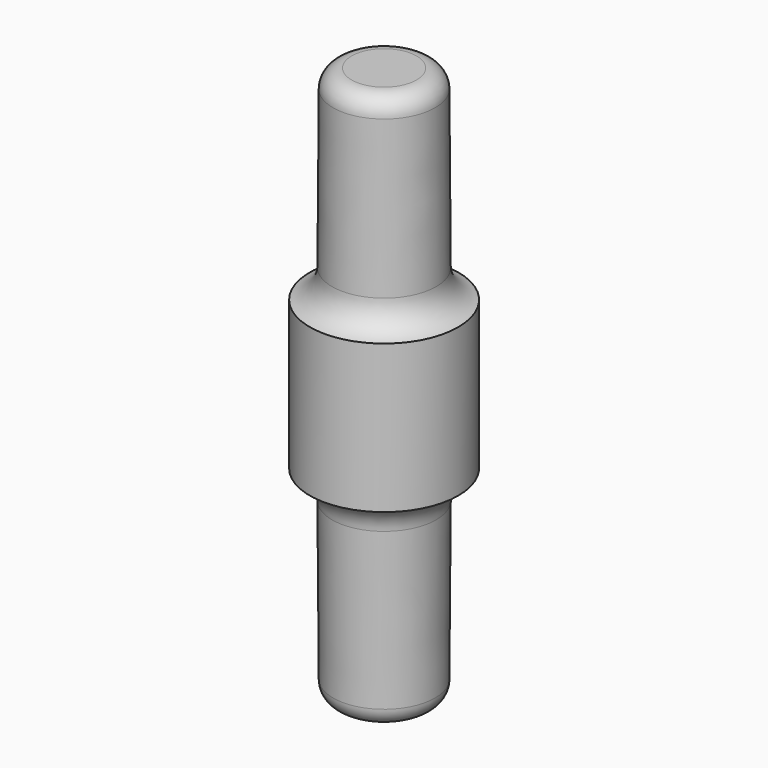
from build123d import *

# Parameters (mm, degrees)
F0_R     = 2.85
F1_DEPTH = 15
F1_TAPER = 0.4
F2_DEPTH = 15
F2_TAPER = 0.4
F0_R_2   = 4
F3_DEPTH = 4
F4_DEPTH = 4
F5_R     = 1
F6_R     = 2.1
F7_DEPTH = 4.2
F8_DEPTH = 2.8


# Not quite as in the source:
# - a fillet or chamfer that OpenCascade refuses, or shapes differently, is made with other operations: its cross-section is extruded or revolved along the edge and cut away or added


with BuildPart() as f1:
    # F0 (on Top) → F1 (new body)
    with BuildSketch(Plane.XY):
        Circle(F0_R)
    extrude(amount=F1_DEPTH, taper=F1_TAPER)

    # F0 (on Top) → F2 (join)
    with BuildSketch(Plane.XY):
        Circle(F0_R)
    extrude(amount=-F2_DEPTH, taper=F2_TAPER)

    # F0 (on Top) → F3 (join)
    with BuildSketch(Plane.XY):
        Circle(F0_R_2)
        Circle(F0_R, mode=Mode.SUBTRACT)
        Circle(F0_R)
    extrude(amount=F3_DEPTH)

    # F0 (on Top) → F4 (join)
    with BuildSketch(Plane.XY):
        Circle(F0_R_2)
        Circle(F0_R, mode=Mode.SUBTRACT)
        Circle(F0_R)
    extrude(amount=-F4_DEPTH)

    # F5
    f5_edges = [f1.edges().sort_by_distance(p)[0] for p in [
        (-2.745279, 0, 15),
        (-2.745279, 0, -15),
    ]]
    fillet(f5_edges, radius=F5_R)

    # F6 (on Front) → F7 (cut)
    with BuildSketch(Plane.XZ):
        Circle(F6_R)
    extrude(amount=-F7_DEPTH, mode=Mode.SUBTRACT)

    # F6 (on Front) → F8 (cut)
    with BuildSketch(Plane.XZ):
        Circle(F6_R)
    extrude(amount=F8_DEPTH, mode=Mode.SUBTRACT)

    # F9: fillet of radius 1.6 on 2 edges, made by hand

    # F9_s1 → F9_t2 (revolve)
    with BuildSketch(Plane.XZ):
        with BuildLine():
            ThreePointArc((4, -4), (3.1462448766, -4.5666406221), (2.8113573865, -5.5350567384))
            Line((2.8113573865, -5.5350567384), (2.7793581663, -5.5348333381))
            Line((2.7793581663, -5.5348333381), (2.7900750581, -3.9997765997))
            Line((2.7900750581, -3.9997765997), (2.8220742783, -3.968))
            ThreePointArc((2.8220742783, -3.968), (3.4110371391, -3.968), (3.9917736321, -3.9690754649))
            Line((3.9917736321, -3.9690754649), (4, -4))
        make_face()
    revolve(axis=Axis((0, 0, -4), (0, 0, -1)))

    # F9_s3 → F9_t4 (revolve)
    with BuildSketch(Plane.XZ):
        with BuildLine():
            ThreePointArc((2.8113573865, 5.5350567384), (3.1462448766, 4.5666406221), (4, 4))
            Line((4, 4), (3.9917736321, 3.9690754649))
            ThreePointArc((3.9917736321, 3.9690754649), (3.4110371391, 3.968), (2.8220742783, 3.968))
            Line((2.8220742783, 3.968), (2.7900750581, 3.9997765997))
            Line((2.7900750581, 3.9997765997), (2.7793581663, 5.5348333381))
            Line((2.7793581663, 5.5348333381), (2.8113573865, 5.5350567384))
        make_face()
    revolve(axis=Axis((0, 0, 4), (0, 0, 1)))


solid = f1.part
